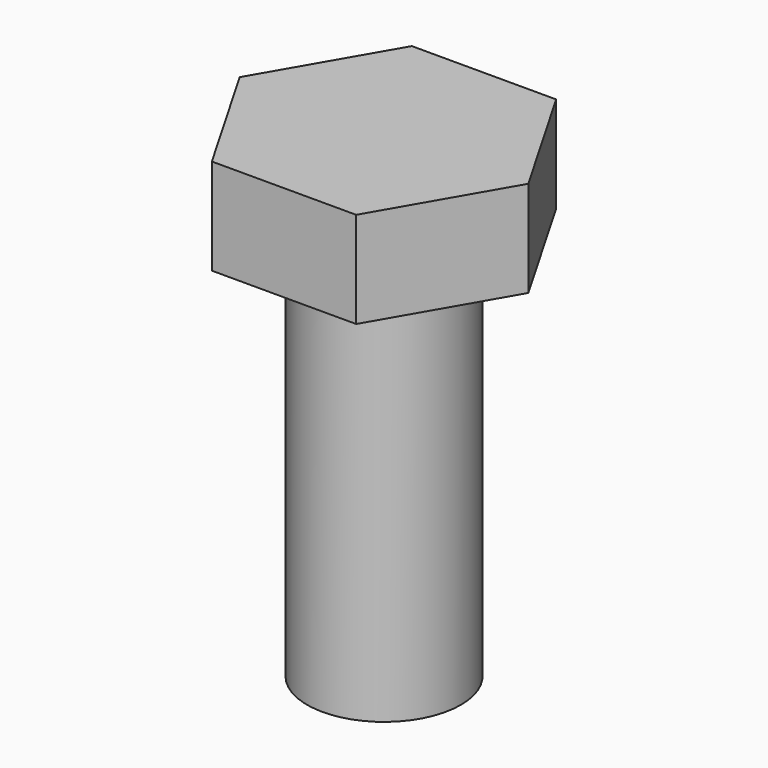
from build123d import *

# Parameters (mm, degrees)
F0_R     = 12.7
F1_DEPTH = 63.5
F3_DEPTH = 15.875


# Not quite as in the source:
# - a feature names something its author has since deleted; it is built from what else it names


with BuildPart() as f1:
    # F0 (on Top) → F1 (new body)
    with BuildSketch(Plane.XY):
        Circle(F0_R)
    extrude(amount=-F1_DEPTH)

    # F2 (on face) → F3 (join)
    with BuildSketch(Plane.XY):
        Polygon((11.9150661804, 20.6375), (-11.9150661804, 20.6375), (-23.8301323608, 0), (-11.9150661804, -20.6375), (11.9150661804, -20.6375), (23.8301323608, 0), align=None)
    extrude(amount=F3_DEPTH)


solid = f1.part
